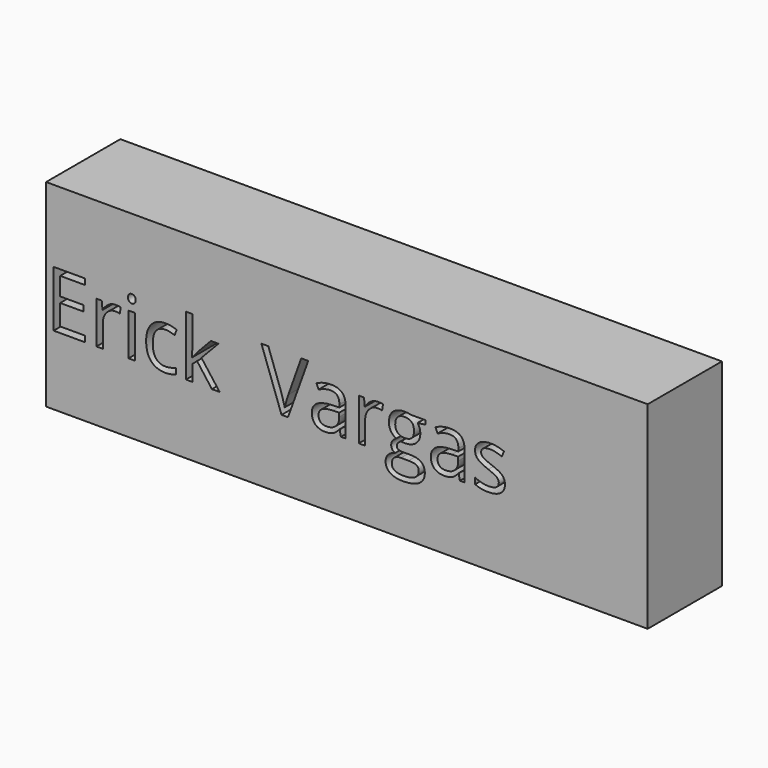
from build123d import *

# Parameters (mm, degrees)
F0_W         = 164.6248847246
F0_H         = 54.1074834764
F1_DEPTH     = 25.4
F2_TEXT_SIZE = 21.5351190949
F3_DEPTH     = 12.7


# Not quite as in the source:
# - Text() gives the source's letters only with a copy of the font that has no kerning and outlines rounded to 1/6400 em; it was checked with that copy


with BuildPart() as f1:
    # F0 (on Front) → F1 (new body)
    with BuildSketch(Plane.XZ):
        Rectangle(F0_W, F0_H)
    extrude(amount=F1_DEPTH)

    # F2 (on face) → F3 (cut)
    with BuildSketch(Plane.XZ.offset(25.4)):
        with Locations((-82.3532911724, -8.0829555647)):
            Text('Erick  Vargas', F2_TEXT_SIZE, font='Open Sans', text_align=(TextAlign.LEFT, TextAlign.BOTTOM))
    extrude(amount=-F3_DEPTH, mode=Mode.SUBTRACT)


solid = f1.part
